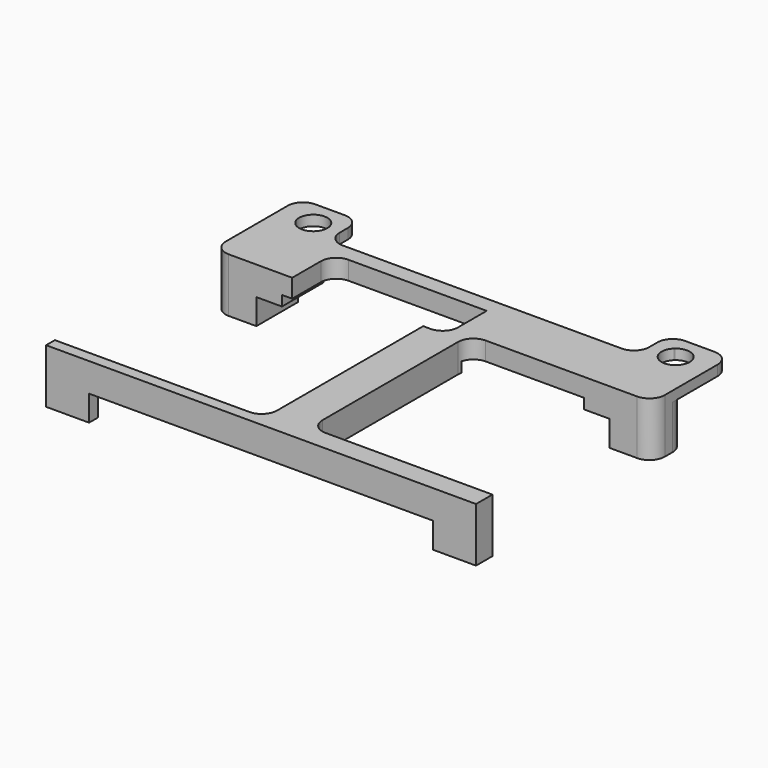
from build123d import *

# Parameters (mm, degrees)
F0_W     = 4.2
F0_H     = 26.5
F0_W_2   = 23.9
F0_H_2   = 1.5
F1_DEPTH = 1
F2_DEPTH = 1.8
F3_DEPTH = 4.3
F4_W     = 17.8
F4_H     = 19.55
F4_W_2   = 30.25
F4_H_2   = 4
F4_W_3   = 42
F4_H_3   = 1
F5_DEPTH = 5.301
F7_DEPTH = 1
F8_R     = 1.5


with BuildPart() as f1:
    # F0 (on Top) → F1 (new body)
    with BuildSketch(Plane.XY):
        with Locations((18.9, -2.75)):
            Rectangle(F0_W, F0_H)
        Polygon((-16.8, -16), (16.8, -16), (16.8, 10.5), (14.3, 10.5), (14.3, 14.5), (11.95, 14.5), (-11.95, 14.5), (-14.3, 14.5), (-14.3, 10.5), (-16.8, 10.5), align=None)
        with BuildLine():
            Line((16.8, 10.5), (21, 10.5))
            Line((21, 10.5), (21, 16))
            Line((21, 16), (16.8, 16))
            Line((16.8, 16), (16.8, 14.5395311443))
            ThreePointArc((16.8, 14.5395311443), (18.2714564725, 14.7506248438), (19.075, 13.5))
            ThreePointArc((19.075, 13.5), (18.2714564725, 12.2493751562), (16.8, 12.4604688557))
            Line((16.8, 12.4604688557), (16.8, 10.5))
        make_face()
        with Locations((-18.9, -2.75)):
            Rectangle(F0_W, F0_H)
        with BuildLine():
            Line((14.3, 10.5), (16.8, 10.5))
            Line((16.8, 10.5), (16.8, 12.4604688557))
            ThreePointArc((16.8, 12.4604688557), (16.3253159421, 13.4705255898), (16.7562706956, 14.5))
            Line((16.7562706956, 14.5), (14.3, 14.5))
            Line((14.3, 14.5), (14.3, 10.5))
        make_face()
        with BuildLine():
            Line((-21, 10.5), (-16.8, 10.5))
            Line((-16.8, 10.5), (-16.8, 12.4604688557))
            ThreePointArc((-16.8, 12.4604688557), (-19.075, 13.5), (-16.8, 14.5395311443))
            Line((-16.8, 14.5395311443), (-16.8, 16))
            Line((-16.8, 16), (-21, 16))
            Line((-21, 16), (-21, 10.5))
        make_face()
        with BuildLine():
            Line((-16.8, 12.4604688557), (-16.8, 10.5))
            Line((-16.8, 10.5), (-14.3, 10.5))
            Line((-14.3, 10.5), (-14.3, 14.5))
            Line((-14.3, 14.5), (-16.7562706956, 14.5))
            ThreePointArc((-16.7562706956, 14.5), (-16.4374128162, 14.044516853), (-16.325, 13.5))
            ThreePointArc((-16.325, 13.5), (-16.4493751562, 12.9285435275), (-16.8, 12.4604688557))
        make_face()
        with BuildLine():
            Line((16.8, 14.5395311443), (16.8, 16))
            Line((16.8, 16), (11.95, 16))
            Line((11.95, 16), (11.95, 14.5))
            Line((11.95, 14.5), (14.3, 14.5))
            Line((14.3, 14.5), (16.7562706956, 14.5))
            ThreePointArc((16.7562706956, 14.5), (16.7779234767, 14.5199999437), (16.8, 14.5395311443))
        make_face()
        with Locations((0, 15.25)):
            Rectangle(F0_W_2, F0_H_2)
        with BuildLine():
            Line((-16.8, 16), (-16.8, 14.5395311443))
            ThreePointArc((-16.8, 14.5395311443), (-16.7779234767, 14.5199999437), (-16.7562706956, 14.5))
            Line((-16.7562706956, 14.5), (-14.3, 14.5))
            Line((-14.3, 14.5), (-11.95, 14.5))
            Line((-11.95, 14.5), (-11.95, 16))
            Line((-11.95, 16), (-16.8, 16))
        make_face()
    extrude(amount=F1_DEPTH)

    # F0 (on Top) → F2 (join)
    with BuildSketch(Plane.XY):
        with Locations((18.9, -2.75)):
            Rectangle(F0_W, F0_H)
        Polygon((-16.8, -16), (16.8, -16), (16.8, 10.5), (14.3, 10.5), (14.3, 14.5), (11.95, 14.5), (-11.95, 14.5), (-14.3, 14.5), (-14.3, 10.5), (-16.8, 10.5), align=None)
        with Locations((-18.9, -2.75)):
            Rectangle(F0_W, F0_H)
    extrude(amount=-F2_DEPTH)

    # F0 (on Top) → F3 (join)
    with BuildSketch(Plane.XY):
        with Locations((-18.9, -2.75)):
            Rectangle(F0_W, F0_H)
        with Locations((18.9, -2.75)):
            Rectangle(F0_W, F0_H)
    extrude(amount=-F3_DEPTH)

    # F4 (on face) → F5 (cut, through all)
    with BuildSketch(Plane.XY.offset(1)):
        Polygon((-21, 5.425), (-21, -13.925), (-0.5, -13.925), (-0.5, 5.425), (-13.3, 5.425), align=None)
        with Locations((12.1, -3.225)):
            Rectangle(F4_W, F4_H)
        with Locations((0, 14)):
            Rectangle(F4_W_2, F4_H_2)
        Polygon((-13.3, 5.425), (-0.5, 5.425), (1.7, 5.425), (1.7, 10.425), (-13.3, 10.425), align=None)
        with Locations((0, -15.5)):
            Rectangle(F4_W_3, F4_H_3)
    extrude(amount=-F5_DEPTH, mode=Mode.SUBTRACT)

    # F6 (on face) → F7 (cut)
    with BuildSketch(Plane(origin=(0, 0, -1.8), x_dir=(1, 0, 0), z_dir=(0, 0, -1))):
        Polygon((-13.3, -5.425), (-14.3, -5.425), (-14.3, -10.5), (-14.3, -12), (14.3, -12), (14.3, -10.5), (14.3, -6.55), (3.2, -6.55), (3.2, -5.425), (1.7, -5.425), (1.7, -10.425), (-13.3, -10.425), align=None)
    extrude(amount=-F7_DEPTH, mode=Mode.SUBTRACT)

    # F8
    f8_edges = [f1.edges().sort_by_distance(p)[0] for p in [
        (-21, 16, 0.5),
        (21, 16, 0.5),
        (21, 10.5, -2.15),
        (-21, 10.5, -2.15),
        (-21, 5.425, -1.65),
        (21, 6.55, -1.65),
        (-15.125, 16, 0.5),
        (15.125, 16, 0.5),
        (15.125, 12, 0.5),
        (-15.125, 12, 0.5),
        (3.2, 6.55, 0.1),
        (3.2, -13, -0.4),
        (-0.5, -13.925, -0.4),
        (-13.3, 10.425, 0.1),
        (1.7, 5.425, 0.1),
    ]]
    fillet(f8_edges, radius=F8_R)


solid = f1.part
